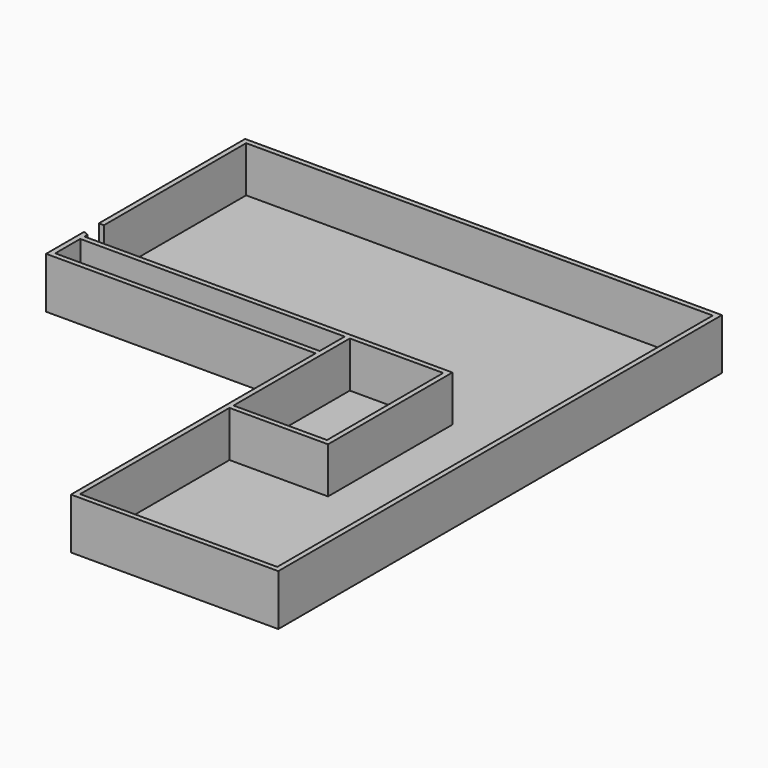
from build123d import *

# Parameters (mm, degrees)
F0_W      = 76.2
F0_H      = 20.32
F0_W_2    = 55.88
F1_DEPTH  = 25
F2_T      = -2.5
F3_W      = 134.58
F3_H      = 20.32
F4_DEPTH  = 22.5
F5_T      = -2.5
F6_W      = 48.3
F6_H      = 76.2
F7_DEPTH  = 25
F8_T      = -2.5
F10_DEPTH = 30


# Not quite as in the source:
# - a shell that OpenCascade refuses in one call is made with other operations: the cavity is built on its own and cut out


with BuildPart() as f1:
    # F0 (on Top) → F1 (new body)
    with BuildSketch(Plane.XY):
        Polygon((-361.3686263561, 74.1551402664), (-361.3686263561, 48.7551402664), (-285.1686263561, 48.7551402664), (-229.2886263561, 48.7551402664), (-178.4886263561, 48.7551402664), (-178.4886263561, -27.4448597336), (-148.0086263561, -27.4448597336), (-148.0086263561, 150.3551402664), (-236.9086263561, 150.3551402664), (-272.4686263561, 150.3551402664), (-361.3686263561, 150.3551402664), align=None)
        with Locations((-323.2686263561, 38.5951402664)):
            Rectangle(F0_W, F0_H)
        with Locations((-257.2286263561, 38.5951402664)):
            Rectangle(F0_W_2, F0_H)
        Polygon((-178.4886263561, 48.7551402664), (-229.2886263561, 48.7551402664), (-229.2886263561, 28.4351402664), (-229.2886263561, -27.4448597336), (-178.4886263561, -27.4448597336), align=None)
        Polygon((-178.4886263561, -27.4448597336), (-229.2886263561, -27.4448597336), (-229.2886263561, -121.4248597336), (-127.6886263561, -121.4248597336), (-127.6886263561, 150.3551402664), (-148.0086263561, 150.3551402664), (-148.0086263561, -27.4448597336), align=None)
    extrude(amount=F1_DEPTH)

    # F2
    f2_openings = [f1.faces().sort_by_distance(p)[0] for p in [
        (-221.527682, 42.066274, 25),
    ]]
    offset(amount=F2_T, openings=f2_openings, kind=Kind.INTERSECTION)

    # F3 (on face) → F4 (join)
    with BuildSketch(Plane.XY.offset(2.5)):
        with Locations((-294.0786263561, 38.5951402664)):
            Rectangle(F3_W, F3_H)
    extrude(amount=F4_DEPTH)

    # F5: a shell. OpenCascade refuses it in one call, so the cavity is built on its own and cut out:
    # the body offset inwards by the wall thickness, plus a prism from it out through each open face.
    f5_core = offset(f1.part, amount=F5_T, kind=Kind.INTERSECTION, mode=Mode.PRIVATE)
    f5_exits = [f5_core.faces().sort_by_distance(p)[0] for p in [
        (-294.078626, 38.59514, 22.5),
    ]]
    add(f5_core, mode=Mode.SUBTRACT)
    extrude(f5_exits, amount=-F5_T, mode=Mode.SUBTRACT)

    # F6 (on Top) → F7 (join)
    with BuildSketch(Plane.XY):
        with Locations((-202.6386263561, 10.6551402664)):
            Rectangle(F6_W, F6_H)
    extrude(amount=F7_DEPTH)

    # F8: a shell. OpenCascade refuses it in one call, so the cavity is built on its own and cut out:
    # the body offset inwards by the wall thickness, plus a prism from it out through each open face.
    f8_core = offset(f1.part, amount=F8_T, kind=Kind.INTERSECTION, mode=Mode.PRIVATE)
    f8_exits = [f8_core.faces().sort_by_distance(p)[0] for p in [
        (-203.888626, 10.65514, 22.5),
    ]]
    add(f8_core, mode=Mode.SUBTRACT)
    extrude(f8_exits, amount=-F8_T, mode=Mode.SUBTRACT)

    # F9 (on Top) → F10 (cut)
    with BuildSketch(Plane.XY):
        Polygon((-358.8686263561, 60.7551402664), (-361.3686263561, 60.7551402664), (-361.3686263561, 51.7551402664), (-358.8686263561, 50.7551402664), align=None)
    extrude(amount=F10_DEPTH, mode=Mode.SUBTRACT)


solid = f1.part
